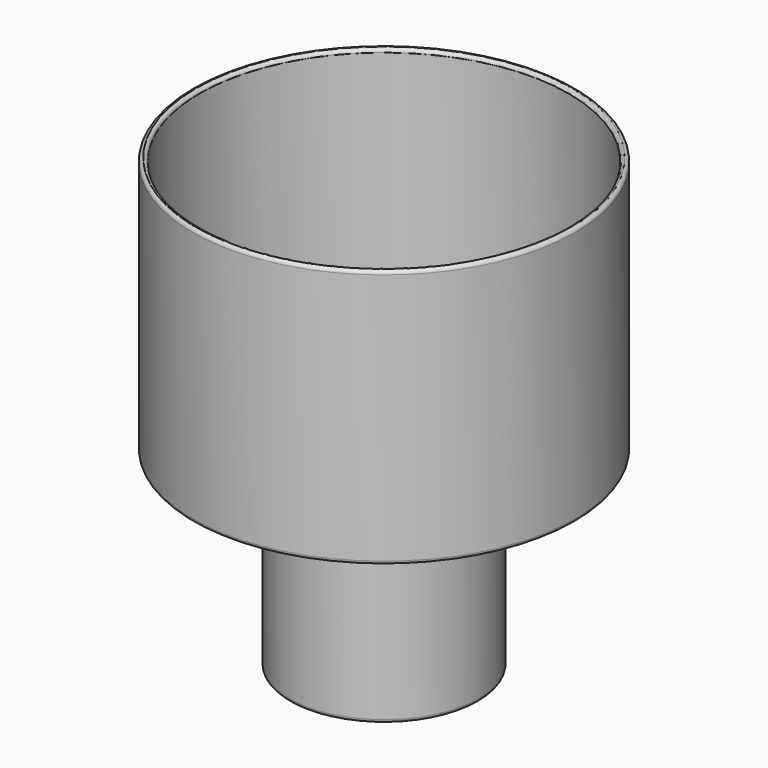
from build123d import *

# Parameters (mm, degrees)
F0_W = 33.02
F0_H = 2.54
F2_R = 1.26999


# Not quite as in the source:
# - a fillet or chamfer is up to 0.001 mm smaller than in the source, because OpenCascade refuses the exact size


with BuildPart() as f1:
    # F0 (on Front) → F1 (revolve)
    with BuildSketch(Plane.XZ):
        Polygon((70.485, 0), (70.485, 95.25), (67.945, 95.25), (67.945, 2.54), (67.945, 0), align=None)
        with Locations((51.435, 1.27)):
            Rectangle(F0_W, F0_H)
        Polygon((34.925, 0), (34.925, 2.54), (32.385, 2.54), (32.385, -69.85), (34.925, -69.85), align=None)
    revolve(axis=Axis((0, 0, -3.7589259446), (0, 0, -1)))

    # F2 (radius 1.27 in the source; OpenCascade refuses exactly that, so slightly less here)
    f2_edges = [f1.edges().sort_by_distance(p)[0] for p in [
        (-67.945, 0, 95.25),
        (-70.485, 0, 95.25),
        (-67.945, 0, 2.54),
        (-70.485, 0, 0),
        (-32.385, 0, -69.85),
        (-32.385, 0, 2.54),
        (-34.925, 0, -69.85),
        (-34.925, 0, 0),
    ]]
    fillet(f2_edges, radius=F2_R)


solid = f1.part
